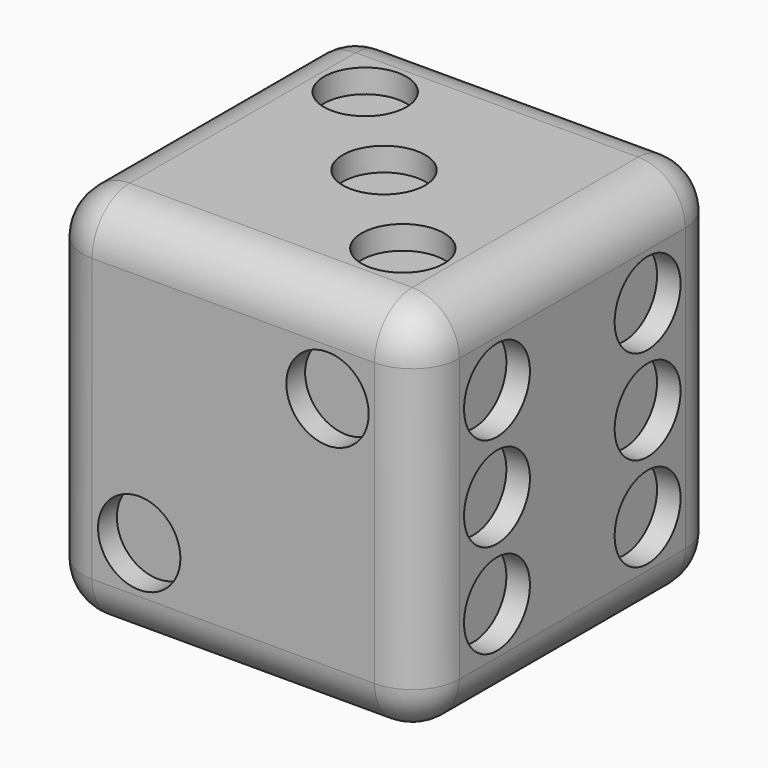
from build123d import *

# Parameters (mm, degrees)
F0_W      = 16
F0_H      = 16
F1_DEPTH  = 16
F2_R      = 1.75
F3_DEPTH  = 1
F4_DEPTH  = 1
F5_R      = 1.75
F6_DEPTH  = 1
F7_R      = 1.75
F8_DEPTH  = 1
F9_R      = 1.75
F10_DEPTH = 1
F11_R     = 1.75
F12_DEPTH = 1
F13_R     = 1.75
F14_DEPTH = 1
F15_R     = 2


# Not quite as in the source:
# - a feature names something its author has since deleted; it is built from what else it names


with BuildPart() as f1:
    # F0 (on Top) → F1 (new body)
    with BuildSketch(Plane.XY):
        Rectangle(F0_W, F0_H)
    extrude(amount=F1_DEPTH)

    # F2 (on face) → F3 (cut)
    with BuildSketch(Plane(origin=(0, 8, 0), x_dir=(-1, 0, 0), z_dir=(0, 1, 0))):
        with Locations((4, 12)):
            Circle(F2_R)
        with Locations((-4, 4)):
            Circle(F2_R)
    extrude(amount=-F3_DEPTH, mode=Mode.SUBTRACT)

    # F2 (on face) → F4 (cut)
    with BuildSketch(Plane(origin=(0, 8, 0), x_dir=(-1, 0, 0), z_dir=(0, 1, 0))):
        with Locations((-4, 12)):
            Circle(F2_R)
        with Locations((0, 8)):
            Circle(F2_R)
        with Locations((4, 4)):
            Circle(F2_R)
    extrude(amount=-F4_DEPTH, mode=Mode.SUBTRACT)

    # F5 (on face) → F6 (cut)
    with BuildSketch(Plane.XZ.offset(8)):
        with Locations((-4, 4)):
            Circle(F5_R)
        with Locations((4, 12)):
            Circle(F5_R)
    extrude(amount=-F6_DEPTH, mode=Mode.SUBTRACT)

    # F7 (on face) → F8 (cut)
    with BuildSketch(Plane.XY.offset(16)):
        Circle(F7_R)
        with Locations((4, -4)):
            Circle(F7_R)
        with Locations((-4, 4)):
            Circle(F7_R)
    extrude(amount=-F8_DEPTH, mode=Mode.SUBTRACT)

    # F9 (on face) → F10 (cut)
    with BuildSketch(Plane.YZ.offset(8)):
        with Locations((-4, 12)):
            Circle(F9_R)
        with Locations((-4, 4)):
            Circle(F9_R)
        with Locations((4, 4)):
            Circle(F9_R)
        with Locations((4, 8)):
            Circle(F9_R)
        with Locations((4, 12)):
            Circle(F9_R)
        with Locations((-4, 8)):
            Circle(F9_R)
    extrude(amount=-F10_DEPTH, mode=Mode.SUBTRACT)

    # F11 (on face) → F12 (cut)
    with BuildSketch(Plane(origin=(0, 0, 0), x_dir=(1, 0, 0), z_dir=(0, 0, -1))):
        with Locations((4, -4)):
            Circle(F11_R)
        with Locations((-4, 4)):
            Circle(F11_R)
        with Locations((4, 4)):
            Circle(F11_R)
        with Locations((-4, -4)):
            Circle(F11_R)
    extrude(amount=-F12_DEPTH, mode=Mode.SUBTRACT)

    # F13 (on face) → F14 (cut)
    with BuildSketch(Plane(origin=(-8, 0, 0), x_dir=(0, -1, 0), z_dir=(-1, 0, 0))):
        with Locations((0, 8)):
            Circle(F13_R)
    extrude(amount=-F14_DEPTH, mode=Mode.SUBTRACT)

    # F15
    f15_edges = [f1.edges().sort_by_distance(p)[0] for p in [
        (8, 0, 16),
        (0, 8, 16),
        (-8, 0, 16),
        (0, -8, 16),
        (-8, -8, 8),
        (-8, 8, 8),
        (-8, 0, 0),
        (0, -8, 0),
        (8, -8, 8),
        (8, 0, 0),
        (8, 8, 8),
        (0, 8, 0),
    ]]
    fillet(f15_edges, radius=F15_R)


solid = f1.part
